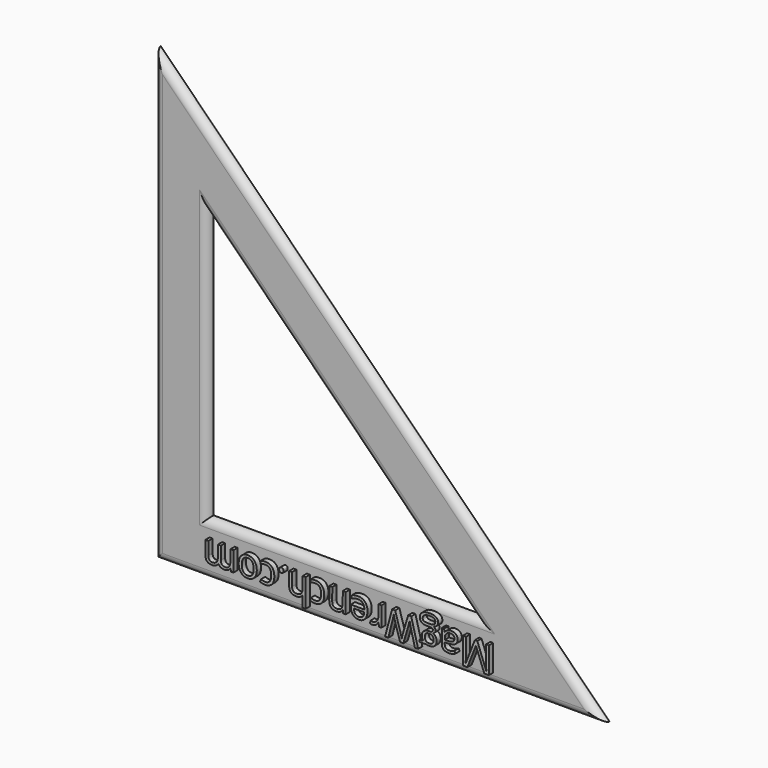
from build123d import *

# Parameters (mm, degrees)
F1_DEPTH     = 3
F2_R         = 2.99999
F3_TEXT_SIZE = 13.947776298
F4_DEPTH     = 2


# Not quite as in the source:
# - a fillet or chamfer is up to 0.001 mm smaller than in the source, because OpenCascade refuses the exact size
# - Text() gives the source's letters only with a copy of the font that has no kerning and outlines rounded to 1/6400 em; it was checked with that copy


with BuildPart() as f1:
    # F0 (on Front) → F1 (new body)
    with BuildSketch(Plane.XZ):
        Polygon((-20, 150), (-20, -20), (150, -20), align=None)
        Polygon((0, 0), (0, 101.7157287525), (101.7157287525, 0), align=None, mode=Mode.SUBTRACT)
    extrude(amount=F1_DEPTH)

    # F2 (radius 3 in the source; OpenCascade refuses exactly that, so slightly less here)
    f2_edges = [f1.edges().sort_by_distance(p)[0] for p in [
        (-20, -3, 65),
        (65, -3, -20),
        (65, -3, 65),
        (0, -3, 50.857864),
        (50.857864, -3, 50.857864),
        (50.857864, -3, 0),
    ]]
    fillet(f2_edges, radius=F2_R)

    # F3 (on face) → F4 (join)
    with BuildSketch(Plane.XZ.offset(3)):
        with Locations(Location((109.7076418587, -6.115482049), (0, 0, 179.8581780978))):
            Text('MagWrench.com', F3_TEXT_SIZE, font='Open Sans', text_align=(TextAlign.LEFT, TextAlign.BOTTOM))
    extrude(amount=F4_DEPTH)


solid = f1.part
